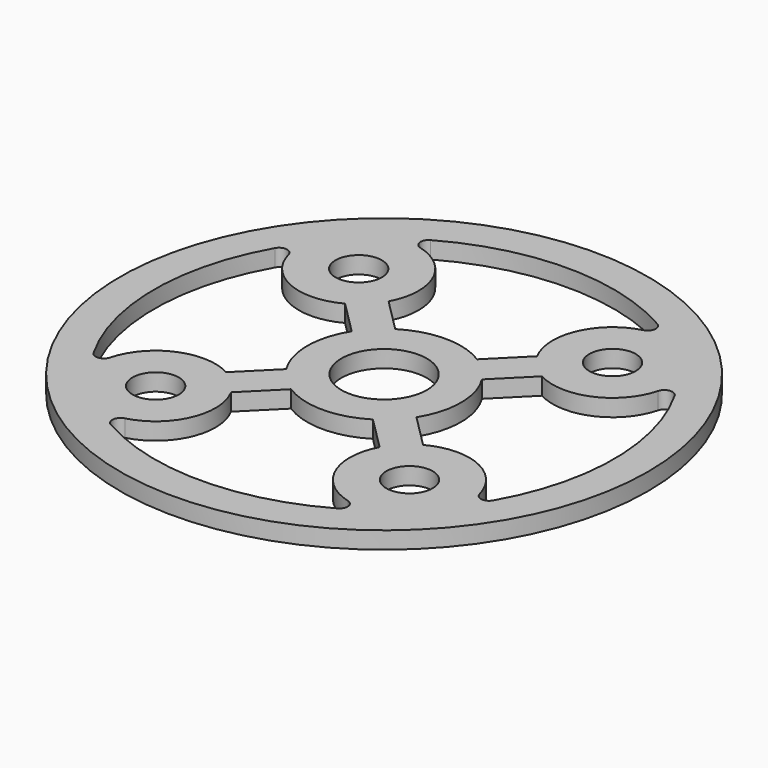
from build123d import *

# Parameters (mm, degrees)
F0_R            = 24.51608
F0_R_2          = 2.15265
F0_R_3          = 3.96875
F1_DEPTH        = 1.5875
F3_DEPTH        = 1.5875
F3_COPIES_COUNT = 4
F4_R            = 0.762


# Not quite as in the source:
# - a pattern or mirror of a feature is missing from the dataset's text; its kind, count and spacing are read off the source's solid


with BuildPart() as f1:
    # F0 (on Top) → F1 (new body)
    with BuildSketch(Plane.XY):
        Circle(F0_R)
        with Locations((-11.7865906, -11.7865906)):
            Circle(F0_R_2, mode=Mode.SUBTRACT)
        with Locations((11.7865906, -11.7865906)):
            Circle(F0_R_2, mode=Mode.SUBTRACT)
        with Locations((-11.7865906, 11.7865906)):
            Circle(F0_R_2, mode=Mode.SUBTRACT)
        Circle(F0_R_3, mode=Mode.SUBTRACT)
        with Locations((11.7865906, 11.7865906)):
            Circle(F0_R_2, mode=Mode.SUBTRACT)
    extrude(amount=F1_DEPTH)

    # F2 (on face) → F3 (cut, through all)
    with BuildSketch(Plane.XY.offset(1.5875)):
        with BuildLine():
            ThreePointArc((-12.5005198818, 17.2967828873), (-7.207099086, 14.9330444032), (-6.8989717457, 9.144035776))
            Line((-6.8989717457, 9.144035776), (-3.8025572131, 6.0476212434))
            ThreePointArc((-3.8025572131, 6.0476212434), (0, 7.14375), (3.8025572131, 6.0476212434))
            Line((3.8025572131, 6.0476212434), (6.8989717457, 9.144035776))
            ThreePointArc((6.8989717457, 9.144035776), (7.207099086, 14.9330444032), (12.5005198818, 17.2967828873))
            ThreePointArc((12.5005198818, 17.2967828873), (0, 21.34108), (-12.5005198818, 17.2967828873))
        make_face()
    f3 = extrude(amount=-F3_DEPTH, mode=Mode.SUBTRACT)

    # F3_copies: F3 ×4 about axis
    f3_copies_axis = Axis((0, 0, 0), (0, 0, 1))
    for i in range(1, F3_COPIES_COUNT):
        add(f3.rotate(f3_copies_axis, i * 360 / F3_COPIES_COUNT), mode=Mode.SUBTRACT)

    # F4
    f4_edges = [f1.edges().sort_by_distance(p)[0] for p in [
        (-12.50052, 17.296783, 0.79375),
        (12.50052, 17.296783, 0.79375),
        (12.50052, -17.296783, 0.79375),
        (-12.50052, -17.296783, 0.79375),
        (17.296783, 12.50052, 0.79375),
        (17.296783, -12.50052, 0.79375),
        (-17.296783, -12.50052, 0.79375),
        (-17.296783, 12.50052, 0.79375),
    ]]
    fillet(f4_edges, radius=F4_R)


solid = f1.part
